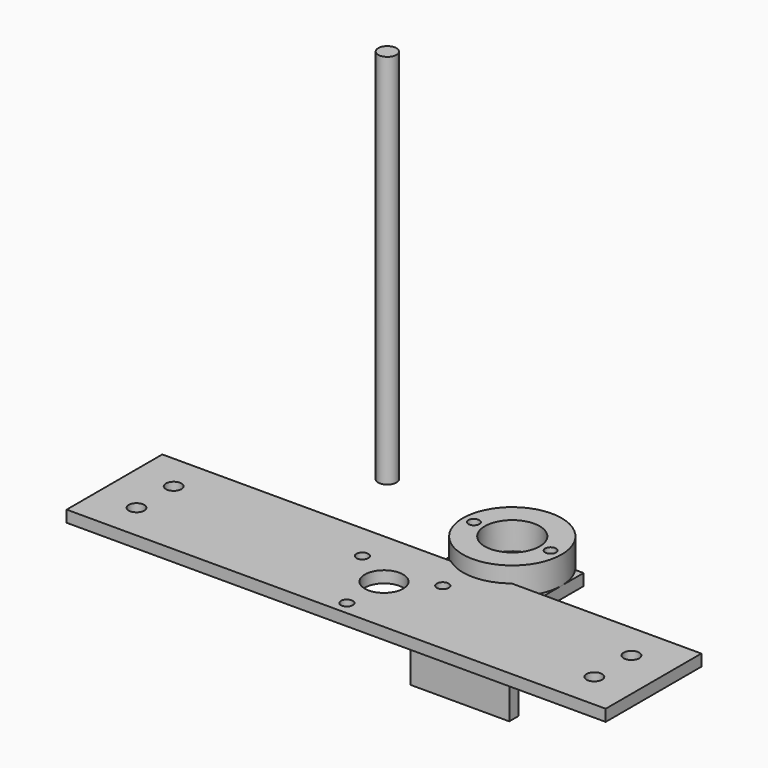
from build123d import *

# Parameters (mm, degrees)
F1_R      = 27
F1_R_2    = 3
F1_R_3    = 15
F2_DEPTH  = 15
F3_R      = 5
F4_DEPTH  = 206
F6_DEPTH  = 54
F7_R      = 3.25
F8_DEPTH  = 25
F9_R      = 4.25
F10_DEPTH = 25
F0_W      = 294.9
F0_H      = 65.4
F0_R      = 3.25
F0_R_2    = 4.25
F0_R_3    = 10.5
F11_DEPTH = 6.35


# Not quite as in the source:
# - a length typed as a fraction of an inch, garbled in the dataset ("3 / 203.2 mm" for 3/8 in), is restored


with BuildPart() as f2:
    # F1 (on Top) → F2 (new body)
    with BuildSketch(Plane.XY):
        with Locations((27, 53.9568550885)):
            Circle(F1_R)
        with Locations((6, 53.9568550885)):
            Circle(F1_R_2, mode=Mode.SUBTRACT)
        with Locations((27, 53.9568550885)):
            Circle(F1_R_3, mode=Mode.SUBTRACT)
        with Locations((48, 53.9568550885)):
            Circle(F1_R_2, mode=Mode.SUBTRACT)
    extrude(amount=F2_DEPTH)


with BuildPart() as f4:
    # F3 (on Top) → F4 (new body)
    with BuildSketch(Plane.XY):
        with Locations((-65.662227571, 84.3633785844)):
            Circle(F3_R)
    extrude(amount=F4_DEPTH)


with BuildPart() as f6:
    # F5 (on Right) → F6 (new body)
    with BuildSketch(Plane.YZ):
        Polygon((68.9568550885, -6.35), (68.9568550885, 0), (18.1568550885, 0), (18.1568550885, -50.8), (24.5068550885, -50.8), (24.5068550885, -6.35), align=None)
    extrude(amount=F6_DEPTH)

    # F7 (on face) → F8 (cut)
    with BuildSketch(Plane.XY):
        with Locations((6, 53.9568550885)):
            Circle(F7_R)
        with Locations((48, 53.9568550885)):
            Circle(F7_R)
    extrude(amount=-F8_DEPTH, mode=Mode.SUBTRACT)

    # F9 (on face) → F10 (cut)
    with BuildSketch(Plane.XZ.offset(-18.1568550885)):
        with Locations((14.3, -28.575)):
            Circle(F9_R)
        with Locations((39.7, -28.575)):
            Circle(F9_R)
    extrude(amount=-F10_DEPTH, mode=Mode.SUBTRACT)


with BuildPart() as f11:
    # F0 (on Top) → F11 (new body)
    with BuildSketch(Plane.XY):
        Rectangle(F0_W, F0_H)
        with Locations((0, -25.4034118443)):
            Circle(F0_R, mode=Mode.SUBTRACT)
        with Locations((-125.225, -12.7)):
            Circle(F0_R_2, mode=Mode.SUBTRACT)
        with Locations((125.225, -12.7)):
            Circle(F0_R_2, mode=Mode.SUBTRACT)
        with Locations((-125.225, 12.7)):
            Circle(F0_R_2, mode=Mode.SUBTRACT)
        Circle(F0_R_3, mode=Mode.SUBTRACT)
        with Locations((-22, 12.7017059222)):
            Circle(F0_R, mode=Mode.SUBTRACT)
        with Locations((22, 12.7017059222)):
            Circle(F0_R, mode=Mode.SUBTRACT)
        with Locations((125.225, 12.7)):
            Circle(F0_R_2, mode=Mode.SUBTRACT)
    extrude(amount=F11_DEPTH)


solid = Compound([f2.part, f4.part, f6.part, f11.part])
